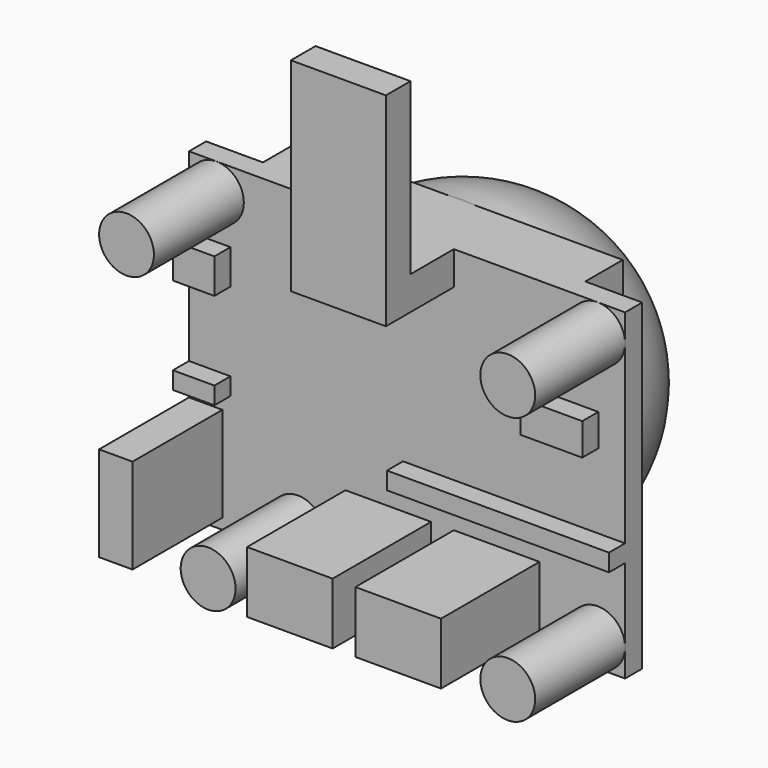
from build123d import *

# Parameters (mm, degrees)
F2_DEPTH  = 1.6
F3_DEPTH  = 5.1
F4_DEPTH  = 17.2
F1_R      = 2.05
F1_W      = 2.5
F1_H      = 7.1
F6_DEPTH  = 8.4
F1_W_2    = 6.4
F1_H_2    = 4.6
F7_DEPTH  = 9.2
F1_W_3    = 3.1
F1_H_3    = 1.3
F1_W_4    = 4.6
F1_H_4    = 2.4
F1_W_5    = 16.6
F1_H_5    = 2.6
F8_DEPTH  = 1.5
F1_W_6    = 7.1
F1_H_6    = 2.5
F9_DEPTH  = 6.35
F10_W     = 7.1
F10_H     = 2.3
F11_DEPTH = 12.7


# Not quite as in the source:
# - a fillet or chamfer that OpenCascade refuses, or shapes differently, is made with other operations: its cross-section is extruded or revolved along the edge and cut away or added


with BuildPart() as f2:
    # F0 (on Front) → F2 (new body)
    with BuildSketch(Plane.XZ):
        Polygon((16.3, -12.05), (16.3, 12.05), (12.05, 12.05), (12.05, 0), (12.05, -12.05), align=None)
        with BuildLine():
            Line((12.05, 0), (12.05, 12.05))
            Line((12.05, 12.05), (0, 12.05))
            ThreePointArc((0, 12.05), (8.5206367133, 8.5206367133), (12.05, 0))
        make_face()
        with BuildLine():
            ThreePointArc((-12.05, 0), (-8.5206367133, 8.5206367133), (0, 12.05))
            Line((0, 12.05), (-12.05, 12.05))
            Line((-12.05, 12.05), (-12.05, 0))
        make_face()
        with BuildLine():
            ThreePointArc((12.05, 0), (8.5206367133, 8.5206367133), (0, 12.05))
            ThreePointArc((0, 12.05), (-8.5206367133, 8.5206367133), (-12.05, 0))
            ThreePointArc((-12.05, 0), (-8.5206367125, -8.5206367141), (2.1e-09, -12.05))
            ThreePointArc((2.1e-09, -12.05), (8.5206367141, -8.5206367125), (12.05, 0))
        make_face()
        with BuildLine():
            Line((12.05, -12.05), (12.05, 0))
            ThreePointArc((12.05, 0), (8.5206367141, -8.5206367125), (2.1e-09, -12.05))
            Line((2.1e-09, -12.05), (12.05, -12.05))
        make_face()
        Polygon((-12.05, 0), (-12.05, 12.05), (-16.3, 12.05), (-16.3, -12.05), (-12.05, -12.05), align=None)
        with BuildLine():
            ThreePointArc((2.1e-09, -12.05), (-8.5206367125, -8.5206367141), (-12.05, 0))
            Line((-12.05, 0), (-12.05, -12.05))
            Line((-12.05, -12.05), (2.1e-09, -12.05))
        make_face()
    extrude(amount=-F2_DEPTH)

    # F0 (on Front) → F3 (join)
    with BuildSketch(Plane.XZ):
        with BuildLine():
            ThreePointArc((2.1e-09, -12.05), (-8.5206367125, -8.5206367141), (-12.05, 0))
            Line((-12.05, 0), (-12.05, -12.05))
            Line((-12.05, -12.05), (2.1e-09, -12.05))
        make_face()
        with BuildLine():
            ThreePointArc((-12.05, 0), (-8.5206367133, 8.5206367133), (0, 12.05))
            Line((0, 12.05), (-12.05, 12.05))
            Line((-12.05, 12.05), (-12.05, 0))
        make_face()
        with BuildLine():
            ThreePointArc((12.05, 0), (8.5206367133, 8.5206367133), (0, 12.05))
            ThreePointArc((0, 12.05), (-8.5206367133, 8.5206367133), (-12.05, 0))
            ThreePointArc((-12.05, 0), (-8.5206367125, -8.5206367141), (2.1e-09, -12.05))
            ThreePointArc((2.1e-09, -12.05), (8.5206367141, -8.5206367125), (12.05, 0))
        make_face()
        with BuildLine():
            Line((12.05, 0), (12.05, 12.05))
            Line((12.05, 12.05), (0, 12.05))
            ThreePointArc((0, 12.05), (8.5206367133, 8.5206367133), (12.05, 0))
        make_face()
        with BuildLine():
            Line((12.05, -12.05), (12.05, 0))
            ThreePointArc((12.05, 0), (8.5206367141, -8.5206367125), (2.1e-09, -12.05))
            Line((2.1e-09, -12.05), (12.05, -12.05))
        make_face()
    extrude(amount=-F3_DEPTH)

    # F0 (on Front) → F4 (join)
    with BuildSketch(Plane.XZ):
        with BuildLine():
            ThreePointArc((12.05, 0), (8.5206367133, 8.5206367133), (0, 12.05))
            ThreePointArc((0, 12.05), (-8.5206367133, 8.5206367133), (-12.05, 0))
            ThreePointArc((-12.05, 0), (-8.5206367125, -8.5206367141), (2.1e-09, -12.05))
            ThreePointArc((2.1e-09, -12.05), (8.5206367141, -8.5206367125), (12.05, 0))
        make_face()
    extrude(amount=-F4_DEPTH)

    # F5: fillet of radius 12 on 1 edges, made by hand

    # F5_s1 → F5_t2 (revolve, cut)
    with BuildSketch(Plane.YZ):
        with BuildLine():
            ThreePointArc((5.2, -12.05), (13.6852813742, -8.5352813742), (17.2, -0.05))
            Line((17.2, -0.05), (17.2, -12.05))
            Line((17.2, -12.05), (5.2, -12.05))
        make_face()
    revolve(axis=Axis((0, 17.2, 0), (0, -1, 0)), mode=Mode.SUBTRACT)

    # F1 (on Front) → F6 (join)
    with BuildSketch(Plane.XZ):
        with Locations((-14.25, 10)):
            Circle(F1_R)
        with Locations((14.25, 10)):
            Circle(F1_R)
        with Locations((14.25, -10)):
            Circle(F1_R)
        with Locations((-8.15, -10)):
            Circle(F1_R)
        with Locations((-15.05, -7.7)):
            Rectangle(F1_W, F1_H)
    extrude(amount=F6_DEPTH)

    # F1 (on Front) → F7 (join)
    with BuildSketch(Plane.XZ):
        with Locations((-1.4, -8.75)):
            Rectangle(F1_W_2, F1_H_2)
        with Locations((6.7, -8.75)):
            Rectangle(F1_W_2, F1_H_2)
    extrude(amount=F7_DEPTH)

    # F1 (on Front) → F8 (join)
    with BuildSketch(Plane.XZ):
        with Locations((-14.75, -2.4)):
            Rectangle(F1_W_3, F1_H_3)
        with Locations((12, 3.65)):
            Rectangle(F1_W_4, F1_H_4)
        with Locations((8, -3.8)):
            Rectangle(F1_W_5, F1_H_3)
        with Locations((-14.75, 5.45)):
            Rectangle(F1_W_3, F1_H_5)
    extrude(amount=F8_DEPTH)

    # F1 (on Front) → F9 (join)
    with BuildSketch(Plane.XZ):
        with Locations((-0.05, 10.8)):
            Rectangle(F1_W_6, F1_H_6)
    extrude(amount=F9_DEPTH)

    # F10 (on face) → F11 (join)
    with BuildSketch(Plane.XY.offset(12.05)):
        with Locations((-0.05, -5.2)):
            Rectangle(F10_W, F10_H)
    extrude(amount=F11_DEPTH)


solid = f2.part
